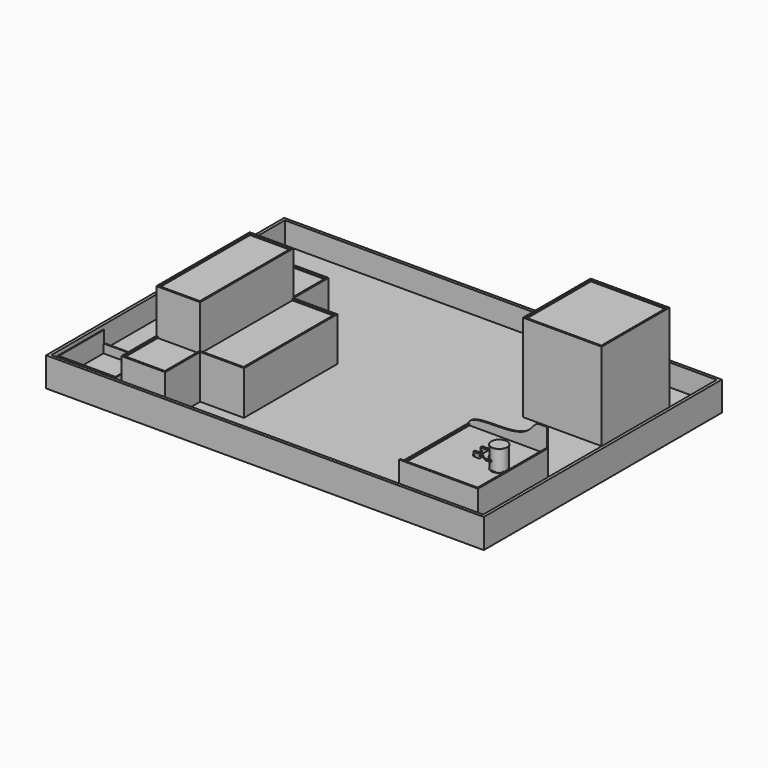
from build123d import *

# Parameters (mm, degrees)
F0_R      = 27.2
F1_DEPTH  = 2.83
F2_R      = 26.4
F3_DEPTH  = 67.36
F4_R      = 27.2
F5_DEPTH  = 2.83
F9_W      = 270
F9_H      = 300
F10_DEPTH = 72
F12_DEPTH = 15
F14_DEPTH = 5
F15_W     = 5
F15_H     = 290
F16_DEPTH = 5
F17_W     = 1500
F17_H     = 1020
F18_DEPTH = 25
F19_W     = 270
F19_H     = 290
F20_DEPTH = 300
F21_W     = 260
F21_H     = 280
F22_DEPTH = 5
F23_W     = 1500
F23_H     = 1020
F23_W_2   = 1480
F23_H_2   = 1000
F24_DEPTH = 75
F26_DEPTH = 150
F27_W     = 150
F27_H     = 400
F28_DEPTH = 150
F29_W     = 140
F29_H     = 390
F30_DEPTH = 5
F31_W     = 140
F31_H     = 145
F31_W_2   = 145
F31_H_2   = 390
F32_DEPTH = 5
F33_R     = 3
F34_DEPTH = 4
F35_R     = 3.99999
F35_2_R   = 3.99999
F36_R     = 3
F37_DEPTH = 8
F38_R     = 3
F39_DEPTH = 8
F40_R     = 3
F40_R_2   = 2.5
F41_DEPTH = 3
F42_R     = 3
F42_R_2   = 2.5
F43_DEPTH = 3
F45_DEPTH = 270.001
F46_W     = 200
F46_H     = 200
F46_W_2   = 194
F46_H_2   = 191
F47_DEPTH = 30
F49_DEPTH = 40
F50_R     = 2.8173532235
F50_R_2   = 2.8078895551
F50_R_3   = 2.8144555676
F50_R_4   = 2.656829774
F51_DEPTH = 6


# Not quite as in the source:
# - a fillet or chamfer is up to 0.001 mm smaller than in the source, because OpenCascade refuses the exact size
# - a feature names something its author has since deleted; it is built from what else it names


with BuildPart() as f1:
    # F0 (on Top) → F1 (new body)
    with BuildSketch(Plane.XY):
        Circle(F0_R)
    extrude(amount=F1_DEPTH)

    # F2 (on face) → F3 (join)
    with BuildSketch(Plane.XY.offset(2.83)):
        Circle(F2_R)
    extrude(amount=F3_DEPTH)

    # F4 (on face) → F5 (join)
    with BuildSketch(Plane.XY.offset(70.19)):
        Circle(F4_R)
    extrude(amount=F5_DEPTH)


with BuildPart() as f10:
    # F9 (on Top) → F10 (new body)
    with BuildSketch(Plane.XY):
        with Locations((-87.8, 0)):
            Rectangle(F9_W, F9_H)
    extrude(amount=-F10_DEPTH)

    # F11 (on face) → F12 (join)
    with BuildSketch(Plane.XY):
        Polygon((-222.8, -145), (-222.8, -150), (47.2, -150), (47.2, 150), (42.2, 150), (42.2, -145), align=None)
    extrude(amount=F12_DEPTH)

    # F13 (on face) → F14 (join)
    with BuildSketch(Plane(origin=(0, 150, 0), x_dir=(-1, 0, 0), z_dir=(0, 1, 0))):
        with BuildLine():
            Line((-21.3134280931, 81.3575685024), (-47.2, 81.3575685024))
            Line((-47.2, 81.3575685024), (-47.2, -72))
            Line((-47.2, -72), (222.8, -72))
            Line((222.8, -72), (222.8, 0))
            add(Edge.make_bspline(
                [(-21.3134280931, 81.3575685024), (-6.3059147253, 81.3822787863), (12.9585432644, 38.1268753575), (103.6097013063, 23.6068887567), (223.0224295336, 30.7718731823), (222.8, 0)],
                knots=[0, 0, 0, 0, 0.2487100673, 0.6151112321, 1, 1, 1, 1], degree=3))
        make_face()
    extrude(amount=-F14_DEPTH)

    # F15 (on face) → F16 (join)
    with BuildSketch(Plane.XY):
        with Locations((-220.3, 0)):
            Rectangle(F15_W, F15_H)
    extrude(amount=F16_DEPTH)

    # F17 (on face) → F18 (join)
    with BuildSketch(Plane(origin=(0, 0, -72), x_dir=(1, 0, 0), z_dir=(0, 0, -1))):
        with Locations((-602.8, -260)):
            Rectangle(F17_W, F17_H)
    extrude(amount=F18_DEPTH)

    # F19 (on face) → F20 (join)
    with BuildSketch(Plane.XY.offset(-72)):
        with Locations((-87.8, 525)):
            Rectangle(F19_W, F19_H)
    extrude(amount=F20_DEPTH)

    # F21 (on face) → F22 (cut)
    with BuildSketch(Plane.XY.offset(228)):
        with Locations((-87.8, 525)):
            Rectangle(F21_W, F21_H)
    extrude(amount=-F22_DEPTH, mode=Mode.SUBTRACT)

    # F23 (on face) → F24 (join)
    with BuildSketch(Plane.XY.offset(-72)):
        with Locations((-602.8, 260)):
            Rectangle(F23_W, F23_H)
        with Locations((-602.8, 260)):
            Rectangle(F23_W_2, F23_H_2, mode=Mode.SUBTRACT)
    extrude(amount=F24_DEPTH)

    # F25 (on face) → F26 (join)
    with BuildSketch(Plane.XY.offset(-72)):
        Polygon((-952.8, 460), (-1102.8, 460), (-1102.8, -240), (-952.8, -240), (-952.8, -90), (-802.8, -90), (-802.8, 310), (-952.8, 310), align=None)
    extrude(amount=F26_DEPTH)

    # F27 (on face) → F28 (join)
    with BuildSketch(Plane.XY.offset(78)):
        with Locations((-1027.8, 110)):
            Rectangle(F27_W, F27_H)
    extrude(amount=F28_DEPTH)

    # F29 (on face) → F30 (cut)
    with BuildSketch(Plane.XY.offset(228)):
        with Locations((-1027.8, 110)):
            Rectangle(F29_W, F29_H)
    extrude(amount=-F30_DEPTH, mode=Mode.SUBTRACT)

    # F31 (on face) → F32 (cut)
    with BuildSketch(Plane.XY.offset(78)):
        with Locations((-1027.8, 382.5)):
            Rectangle(F31_W, F31_H)
        with Locations((-880.3, 110)):
            Rectangle(F31_W_2, F31_H_2)
        with Locations((-1027.8, -162.5)):
            Rectangle(F31_W, F31_H)
    extrude(amount=-F32_DEPTH, mode=Mode.SUBTRACT)

    # F46 (on face) → F47 (join)
    with BuildSketch(Plane.XY.offset(-72)):
        with Locations((-1232.8, -130)):
            Rectangle(F46_W, F46_H)
        with Locations((-1232.8, -128.5)):
            Rectangle(F46_W_2, F46_H_2, mode=Mode.SUBTRACT)
    extrude(amount=F47_DEPTH)

    # F48 (on face) → F49 (join)
    with BuildSketch(Plane.XY.offset(-42)):
        Polygon((-1329.8, -30), (-1332.8, -30), (-1332.8, -230), (-1329.8, -230), (-1135.8, -230), (-1132.8, -230), (-1132.8, -30), (-1135.8, -30), (-1135.8, -224), (-1329.8, -224), align=None)
    extrude(amount=F49_DEPTH)


with BuildPart() as f34:
    # F33 (on offset) → F34 (new body, symmetric)
    with BuildSketch(Plane.XY.offset(25)):
        with BuildLine():
            Line((-55, -12), (-74.5, -12))
            Line((-74.5, -12), (-74.5, -13))
            Line((-74.5, -13), (-65.6457513111, -13))
            ThreePointArc((-65.6457513111, -13), (-67, -16), (-65.6457513111, -19))
            Line((-65.6457513111, -19), (-74.5, -19))
            Line((-74.5, -19), (-74.5, -20))
            Line((-74.5, -20), (-55, -20))
            ThreePointArc((-55, -20), (-51, -16), (-55, -12))
        make_face()
        with Locations((-63, -16)):
            Circle(F33_R, mode=Mode.SUBTRACT)
        with Locations((-55, -16)):
            Circle(F33_R, mode=Mode.SUBTRACT)
    extrude(amount=F34_DEPTH, both=True)

    # F35 (radius 4 in the source; OpenCascade refuses exactly that, so slightly less here)
    f35_edges = [f34.edges().sort_by_distance(p)[0] for p in [
        (-74.5, -19.5, 29),
        (-74.5, -12.5, 29),
        (-74.5, -19.5, 21),
        (-74.5, -12.5, 21),
    ]]
    fillet(f35_edges, radius=F35_R)

    # F36 (on face) → F37 (join, through all)
    with BuildSketch(Plane.XZ.offset(20)):
        with Locations((-70.5, 25)):
            Circle(F36_R)
    extrude(amount=-F37_DEPTH)

    # F42 (on offset) → F43 (join, symmetric)
    with BuildSketch(Plane.XY.offset(25)):
        with Locations((-63, -16)):
            Circle(F42_R)
        with Locations((-63, -16)):
            Circle(F42_R_2, mode=Mode.SUBTRACT)
        with Locations((-55, -16)):
            Circle(F42_R)
        with Locations((-55, -16)):
            Circle(F42_R_2, mode=Mode.SUBTRACT)
    extrude(amount=F43_DEPTH, both=True)


with BuildPart() as f34b:
    # F33 (on offset) → F34, piece 2 (new body, symmetric)
    with BuildSketch(Plane.XY.offset(25)):
        with BuildLine():
            Line((-74.5, 13), (-74.5, 12))
            Line((-74.5, 12), (-55, 12))
            ThreePointArc((-55, 12), (-51, 16), (-55, 20))
            Line((-55, 20), (-74.5, 20))
            Line((-74.5, 20), (-74.5, 19))
            Line((-74.5, 19), (-65.6457513111, 19))
            ThreePointArc((-65.6457513111, 19), (-67, 16), (-65.6457513111, 13))
            Line((-65.6457513111, 13), (-74.5, 13))
        make_face()
        with Locations((-63, 16)):
            Circle(F33_R, mode=Mode.SUBTRACT)
        with Locations((-55, 16)):
            Circle(F33_R, mode=Mode.SUBTRACT)
    extrude(amount=F34_DEPTH, both=True)

    # F35#2 (radius 4 in the source; OpenCascade refuses exactly that, so slightly less here)
    f35_2_edges = [f34b.edges().sort_by_distance(p)[0] for p in [
        (-74.5, 12.5, 29),
        (-74.5, 19.5, 29),
        (-74.5, 19.5, 21),
        (-74.5, 12.5, 21),
    ]]
    fillet(f35_2_edges, radius=F35_2_R)

    # F38 (on face) → F39 (join, through all)
    with BuildSketch(Plane(origin=(0, 20, 0), x_dir=(-1, 0, 0), z_dir=(0, 1, 0))):
        with Locations((70.5, 25)):
            Circle(F38_R)
    extrude(amount=-F39_DEPTH)

    # F40 (on offset) → F41 (join, symmetric)
    with BuildSketch(Plane.XY.offset(25)):
        with Locations((-55, 16)):
            Circle(F40_R)
        with Locations((-55, 16)):
            Circle(F40_R_2, mode=Mode.SUBTRACT)
        with Locations((-63, 16)):
            Circle(F40_R)
        with Locations((-63, 16)):
            Circle(F40_R_2, mode=Mode.SUBTRACT)
    extrude(amount=F41_DEPTH, both=True)


with BuildPart() as f45_tool:
    # F44 (on face) → F45 (new body, through all)
    with BuildSketch(Plane(origin=(0, 20, 0), x_dir=(-1, 0, 0), z_dir=(0, 1, 0))):
        with BuildLine():
            Line((71.5, 26), (71.5, 27.2912878475))
            ThreePointArc((71.5, 27.2912878475), (70.5, 27.5), (69.5, 27.2912878475))
            Line((69.5, 27.2912878475), (69.5, 26))
            Line((69.5, 26), (68.2087121525, 26))
            ThreePointArc((68.2087121525, 26), (68, 25), (68.2087121525, 24))
            Line((68.2087121525, 24), (69.5, 24))
            Line((69.5, 24), (69.5, 22.7087121525))
            ThreePointArc((69.5, 22.7087121525), (70.5, 22.5), (71.5, 22.7087121525))
            Line((71.5, 22.7087121525), (71.5, 24))
            Line((71.5, 24), (72.7912878475, 24))
            ThreePointArc((72.7912878475, 24), (73, 25), (72.7912878475, 26))
            Line((72.7912878475, 26), (71.5, 26))
        make_face()
    extrude(amount=-F45_DEPTH)


with BuildPart() as f34_1:
    add(f34.part)

    # F45: cut by f45_tool
    add(f45_tool.part, mode=Mode.SUBTRACT)


with BuildPart() as f34b_1:
    add(f34b.part)

    # F45: cut by f45_tool
    add(f45_tool.part, mode=Mode.SUBTRACT)


with BuildPart() as f51:
    # F50 (on face) → F51 (new body)
    with BuildSketch(Plane.XY.offset(29)):
        with BuildLine():
            Line((-39.1727497998, 19.9571158737), (-71.1982087493, 19.9571158737))
            ThreePointArc((-71.1982087493, 19.9571158737), (-73.3195290929, 19.0784362173), (-74.1982087493, 16.9571158737))
            Line((-74.1982087493, 16.9571158737), (-74.1982087493, 14.3730141893))
            ThreePointArc((-74.1982087493, 14.3730141893), (-73.3195290929, 12.2516938457), (-71.1982087493, 11.3730141893))
            Line((-71.1982087493, 11.3730141893), (-44.3680129507, 11.3730141893))
            ThreePointArc((-44.3680129507, 11.3730141893), (-46.4962255314, -0.3267408138), (-43.9522635738, -11.9431866333))
            Line((-43.9522635738, -11.9431866333), (-71.0793446674, -11.9431866333))
            ThreePointArc((-71.0793446674, -11.9431866333), (-73.241465529, -12.8634670897), (-74.0770813417, -15.0596977134))
            Line((-74.0770813417, -15.0596977134), (-73.9819935972, -17.5062291378))
            ThreePointArc((-73.9819935972, -17.5062291378), (-73.0508570799, -19.5643821217), (-70.9479562255, -20.3894984262))
            Line((-70.9479562255, -20.3894984262), (-38.7609787285, -20))
            ThreePointArc((-38.7609787285, -20), (-23.0084069826, -29.2826726819), (-4.7845798545, -27.7982018888))
            ThreePointArc((-4.7845798545, -27.7982018888), (-28.383075273, 0.3651769416), (-4.0852902457, 27.9275160283))
            ThreePointArc((-4.0852902457, 27.9275160283), (-22.9422270461, 29.7233429286), (-39.1727497998, 19.9571158737))
        make_face()
        with Locations((-63, -16)):
            Circle(F50_R, mode=Mode.SUBTRACT)
        with Locations((-55, -16)):
            Circle(F50_R_2, mode=Mode.SUBTRACT)
        with Locations((-63.012689352, 16.1359552294)):
            Circle(F50_R_3, mode=Mode.SUBTRACT)
        with Locations((-55, 16)):
            Circle(F50_R_4, mode=Mode.SUBTRACT)
    extrude(amount=F51_DEPTH)


solid = Compound([f1.part, f10.part, f34_1.part, f34b_1.part, f51.part])
